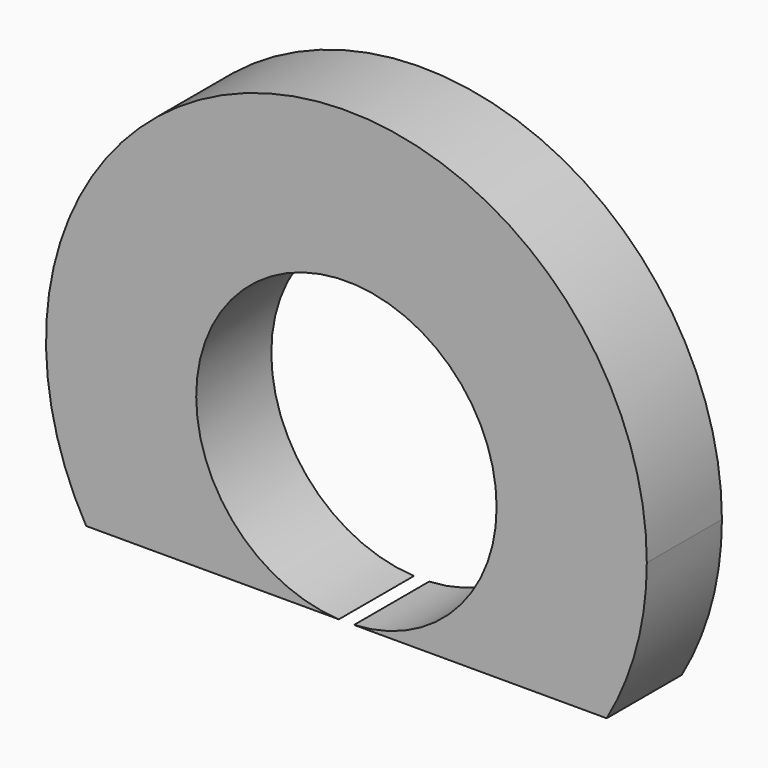
from build123d import *

# Parameters (mm, degrees)
F1_DEPTH = 2.5


# Not quite as in the source:
# - a feature names something its author has since deleted; it is built from what else it names


with BuildPart() as f1:
    # F0 (on Front) → F1 (new body)
    with BuildSketch(Plane.XZ):
        with BuildLine():
            ThreePointArc((-0.2018715048, -3.3093462615), (-2.7561308007, 3.5844774855), (4, 0.6855564776))
            ThreePointArc((4, 0.6855564776), (2.8989210078, -2.070574323), (0.2018715048, -3.3093462615))
            Line((0.2018715048, -3.3093462615), (4.4766898602, -3.3093462615))
            ThreePointArc((4.4766898602, -3.3093462615), (5.6062527218, -1.4521830807), (6, 0.6855564776))
            ThreePointArc((6, 0.6855564776), (-2.1377395584, 6.2918091994), (-4.4766898602, -3.3093462615))
            Line((-4.4766898602, -3.3093462615), (-0.2018715048, -3.3093462615))
        make_face()
        with BuildLine():
            Line((-6.9311436361, -3.3093462615), (-4.4766898602, -3.3093462615))
            ThreePointArc((-4.4766898602, -3.3093462615), (-2.1377395584, 6.2918091994), (6, 0.6855564776))
            ThreePointArc((6, 0.6855564776), (5.6062527218, -1.4521830807), (4.4766898602, -3.3093462615))
            Line((4.4766898602, -3.3093462615), (6.9311436361, -3.3093462615))
            ThreePointArc((6.9311436361, -3.3093462615), (7.7281676059, -1.3821537186), (8, 0.6855564776))
            ThreePointArc((8, 0.6855564776), (-2.0677101962, 8.4137240835), (-6.9311436361, -3.3093462615))
        make_face()
    extrude(amount=F1_DEPTH)


solid = f1.part
